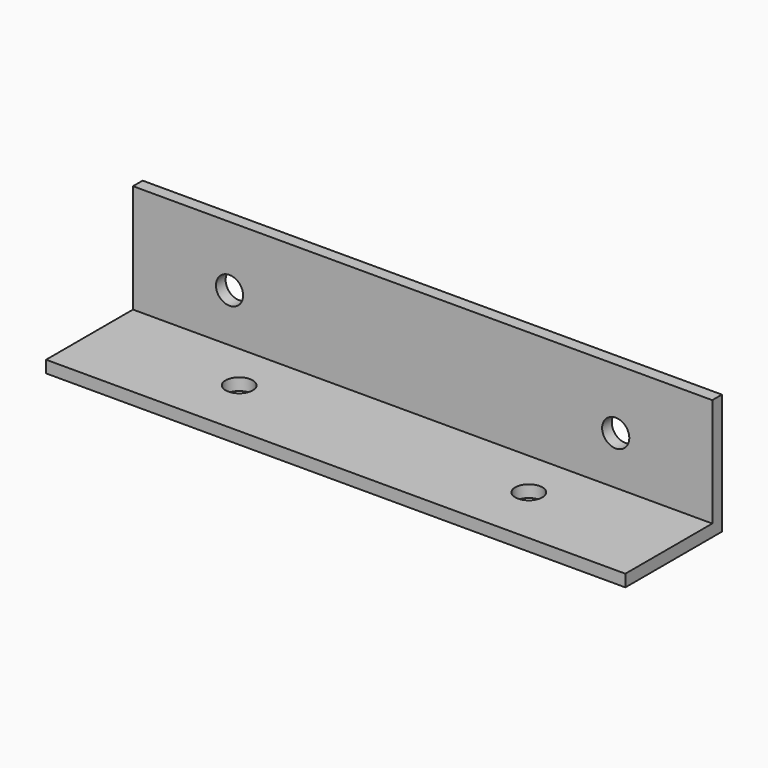
from build123d import *

# Parameters (mm, degrees)
F0_W     = 76.2
F0_H     = 15.875
F1_DEPTH = 0.79375
F2_R     = 1.7859375
F3_DEPTH = 1.5875
F4_W     = 76.2
F4_H     = 1.5875
F5_DEPTH = 14.2875
F6_R     = 1.7859375
F6_R_2   = 1.7907
F7_DEPTH = 1.5875


# Not quite as in the source:
# - a pattern or mirror of a feature is missing from the dataset's text; its kind, count and spacing are read off the source's solid


with BuildPart() as f1:
    # F0 (on Front) → F1 (new body, symmetric)
    with BuildSketch(Plane.XZ):
        Rectangle(F0_W, F0_H)
    extrude(amount=F1_DEPTH, both=True)

    # F2 (on face) → F3 (cut, through all)
    with BuildSketch(Plane.XZ.offset(0.79375)):
        with Locations((-25.4, 0)):
            Circle(F2_R)
    f3 = extrude(amount=-F3_DEPTH, mode=Mode.SUBTRACT)

    # F3_copies: F3 across plane
    add(f3.mirror(Plane(origin=(0, 0, 0), x_dir=(0, 0, 1), z_dir=(1, 0, 0))), mode=Mode.SUBTRACT)

    # F4 (on face) → F5 (join)
    with BuildSketch(Plane.XZ.offset(0.79375)):
        with Locations((0, -7.14375)):
            Rectangle(F4_W, F4_H)
    extrude(amount=F5_DEPTH)

    # F6 (on face) → F7 (cut, through all)
    with BuildSketch(Plane.XY.offset(-6.35)):
        with Locations((-19.05, -7.14375)):
            Circle(F6_R)
        with Locations((19.05, -7.14375)):
            Circle(F6_R_2)
    extrude(amount=-F7_DEPTH, mode=Mode.SUBTRACT)


solid = f1.part
